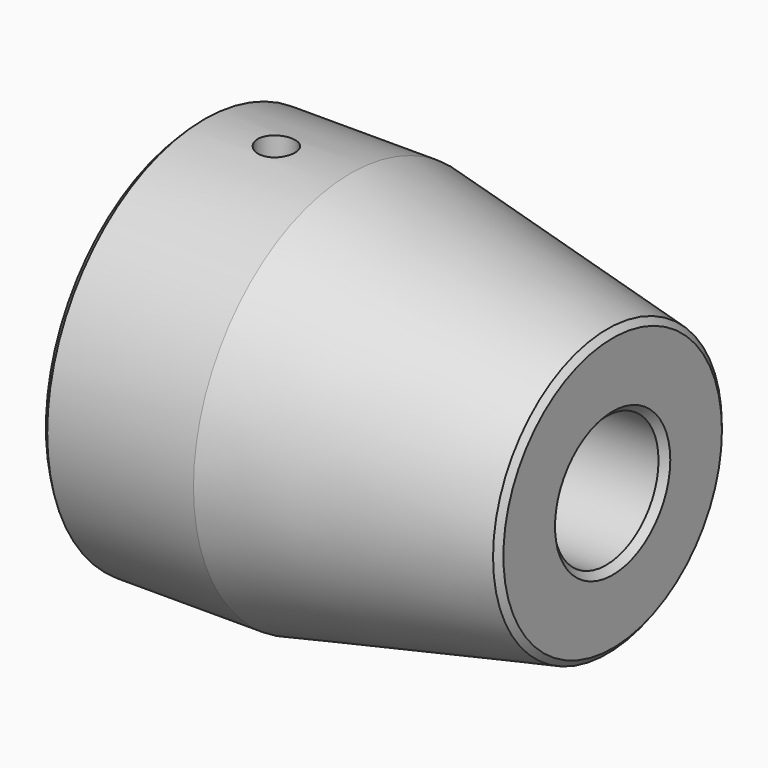
from build123d import *

# Parameters (mm, degrees)
F0_R      = 45
F3_DEPTH  = 35
F4_R      = 45
F2_R      = 32.5
F9_D      = 30
F10_D     = 8.5
F10_DEPTH = 45
F10_START = 0.2011441
F10_TIP   = 2.5536576309


# Not quite as in the source:
# - a fillet or chamfer that OpenCascade refuses, or shapes differently, is made with other operations: its cross-section is extruded or revolved along the edge and cut away or added


with BuildPart() as f3:
    # F0 (on Right) → F3 (new body)
    with BuildSketch(Plane.YZ):
        Circle(F0_R)
    extrude(amount=F3_DEPTH)

    # F4 (on face) → F5 section 0
    with BuildSketch(Plane.YZ.offset(35)):
        Circle(F4_R)
    # F2 (on offset) → F5 section 1
    with BuildSketch(Plane.YZ.offset(95)):
        Circle(F2_R)
    loft()

    # F9 (through all)
    with Locations(Plane.YZ.offset(95)):
        with Locations((0, 0)):
            Hole(F9_D / 2)

    # F10
    # its depths count from where the whole tool has entered the part; down to there all is cleared
    with Locations(Plane.XY.offset(45).offset(-F10_START)):
        with Locations((18, 0)):
            Hole(F10_D / 2, depth=F10_DEPTH)
            with Locations((0, 0, -(F10_DEPTH + F10_TIP / 2))):  # 118° drill point
                Cone(0, F10_D / 2, F10_TIP, mode=Mode.SUBTRACT)

    # F11: chamfer of 1.5 on 4 edges, made by hand

    # F11_s1 → F11_t2 (revolve, cut)
    with BuildSketch(Plane.XY):
        Polygon((93.8059313812, 32.7487642956), (95, 31.280293666), (95, 32.5), align=None)
    revolve(axis=Axis((95, 0, 0), (1, 0, 0)), mode=Mode.SUBTRACT)

    # F11_s3 → F11_t4 (revolve, cut)
    with BuildSketch(Plane.XY):
        Polygon((1.5, 45), (0, 43.5), (0, 45), align=None)
    revolve(axis=Axis((0, 0, 0), (1, 0, 0)), mode=Mode.SUBTRACT)

    # F11_s5 → F11_t6 (revolve, cut)
    with BuildSketch(Plane.XY):
        Polygon((0, 16.5), (1.5, 15), (0, 15), align=None)
    revolve(axis=Axis((0, 0, 0), (1, 0, 0)), mode=Mode.SUBTRACT)

    # F11_s7 → F11_t8 (revolve, cut)
    with BuildSketch(Plane.XY):
        Polygon((93.5, 15), (95, 16.5), (95, 15), align=None)
    revolve(axis=Axis((95, 0, 0), (1, 0, 0)), mode=Mode.SUBTRACT)


solid = f3.part
